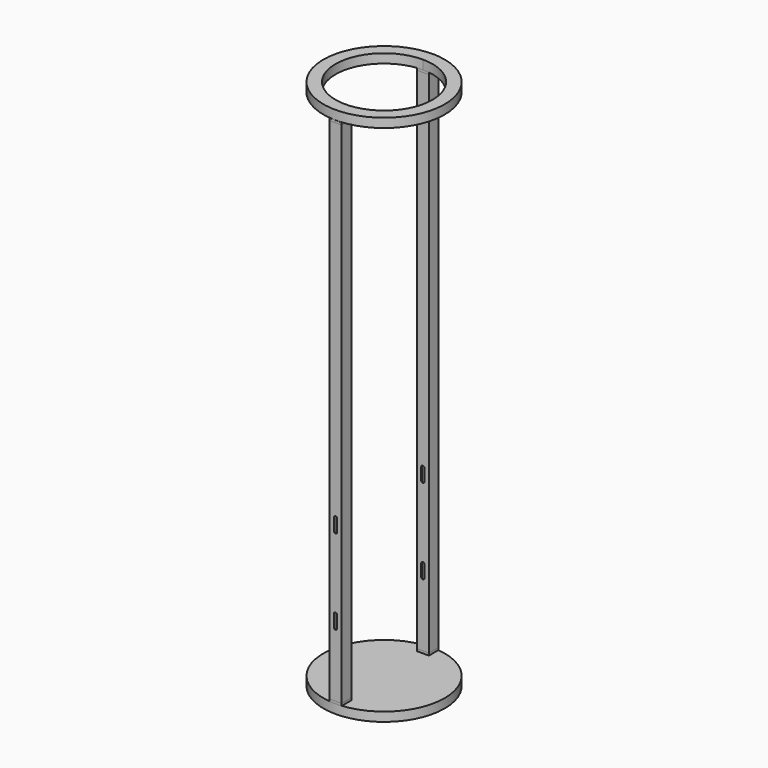
from build123d import *

# Parameters (mm, degrees)
F0_R           = 127
F1_DEPTH       = 19.05
F3_D           = 5.1054
F3_CSINK_D     = 10.4394
F3_CSINK_ANGLE = 82
F5_W           = 25.4
F5_H           = 25.4
F6_DEPTH       = 4.7625
F7_W           = 25.4
F7_H           = 25.4
F7_W_2         = 22.225
F7_H_2         = 22.225
F8_DEPTH       = 1066.8
F13_DEPTH      = 19.05
F15_DEPTH      = 254.001


# Not quite as in the source:
# - a pattern or mirror of a feature is missing from the dataset's text; its kind, count and spacing are read off the source's solid


with BuildPart() as f1:
    # F0 (on Top) → F1 (new body)
    with BuildSketch(Plane.XY):
        Circle(F0_R)
    extrude(amount=F1_DEPTH)

    # F3 (through all)
    with Locations(Plane(origin=(0, 0, 0), x_dir=(1, 0, 0), z_dir=(0, 0, -1))):
        with Locations((0, 114.3)):
            f3 = CounterSinkHole(F3_D / 2, F3_CSINK_D / 2, counter_sink_angle=F3_CSINK_ANGLE)

    # F3_copies: F3 across plane
    add(f3.mirror(Plane.ZX), mode=Mode.SUBTRACT)


with BuildPart() as f6:
    # F5 (on face) → F6 (new body)
    with BuildSketch(Plane.XY.offset(19.05)):
        with Locations((0, 114.3)):
            Rectangle(F5_W, F5_H)
    extrude(amount=F6_DEPTH)


with BuildPart() as f8:
    # F7 (on face) → F8 (new body)
    with BuildSketch(Plane.XY.offset(23.8125)):
        with Locations((0, 114.3)):
            Rectangle(F7_W, F7_H)
        with Locations((0, 114.3)):
            Rectangle(F7_W_2, F7_H_2, mode=Mode.SUBTRACT)
    extrude(amount=F8_DEPTH)


with BuildPart() as f10_1:
    # F10: instance of F6
    add(f6.part.mirror(Plane(origin=(0, 114.3, 557.2125), x_dir=(1, 0, 0), z_dir=(0, 0, -1))))


with BuildPart() as f11_1:
    # F11: instance of F8
    add(f8.part.mirror(Plane.XZ))


with BuildPart() as f11_2:
    # F11: instance of F10_1
    add(f10_1.part.mirror(Plane.XZ))


with BuildPart() as f11_3:
    # F11: instance of F6
    add(f6.part.mirror(Plane.XZ))


with BuildPart() as f13:
    # F12 (on face) → F13 (new body)
    with BuildSketch(Plane.XY.offset(1095.375)):
        with BuildLine():
            ThreePointArc((-12.7, 126.3634045125), (-85.1941899427, -94.1857207861), (127, 0))
            ThreePointArc((127, 0), (94.1857207861, 85.1941899427), (12.7, 126.3634045125))
            Line((12.7, 126.3634045125), (12.7, 101.6))
            Line((12.7, 101.6), (0, 101.6))
            Line((0, 101.6), (-12.7, 101.6))
            Line((-12.7, 101.6), (-12.7, 126.3634045125))
        make_face()
        with BuildLine():
            ThreePointArc((101.6, 0), (-71.8420489686, -71.8420489686), (0, 101.6))
            ThreePointArc((0, 101.6), (71.8420489686, 71.8420489686), (101.6, 0))
        make_face(mode=Mode.SUBTRACT)
        with BuildLine():
            Line((12.7, 101.6), (12.7, 126.3634045125))
            ThreePointArc((12.7, 126.3634045125), (6.3579724326, 126.840751285), (0, 127))
            ThreePointArc((0, 127), (-6.3579724326, 126.840751285), (-12.7, 126.3634045125))
            Line((-12.7, 126.3634045125), (-12.7, 101.6))
            Line((-12.7, 101.6), (0, 101.6))
            Line((0, 101.6), (12.7, 101.6))
        make_face()
    extrude(amount=F13_DEPTH)


with BuildPart() as f15_tool:
    # F14 (on face) → F15 (new body, through all)
    with BuildSketch(Plane.XZ.offset(127)):
        with BuildLine():
            ThreePointArc((3.3782, 361.95), (0, 365.3282), (-3.3782, 361.95))
            Line((-3.3782, 361.95), (-3.3782, 336.55))
            ThreePointArc((-3.3782, 336.55), (0, 333.1718), (3.3782, 336.55))
            Line((3.3782, 336.55), (3.3782, 361.95))
        make_face()
        with BuildLine():
            ThreePointArc((3.3782, 184.15), (0, 187.5282), (-3.3782, 184.15))
            Line((-3.3782, 184.15), (-3.3782, 158.75))
            ThreePointArc((-3.3782, 158.75), (0, 155.3718), (3.3782, 158.75))
            Line((3.3782, 158.75), (3.3782, 184.15))
        make_face()
    extrude(amount=-F15_DEPTH)


with BuildPart() as f8_1:
    add(f8.part)

    # F15: cut by f15_tool
    add(f15_tool.part, mode=Mode.SUBTRACT)


with BuildPart() as f11_1_1:
    add(f11_1.part)

    # F15: cut by f15_tool
    add(f15_tool.part, mode=Mode.SUBTRACT)


solid = Compound([f1.part, f6.part, f10_1.part, f11_2.part, f11_3.part, f13.part, f8_1.part, f11_1_1.part])
